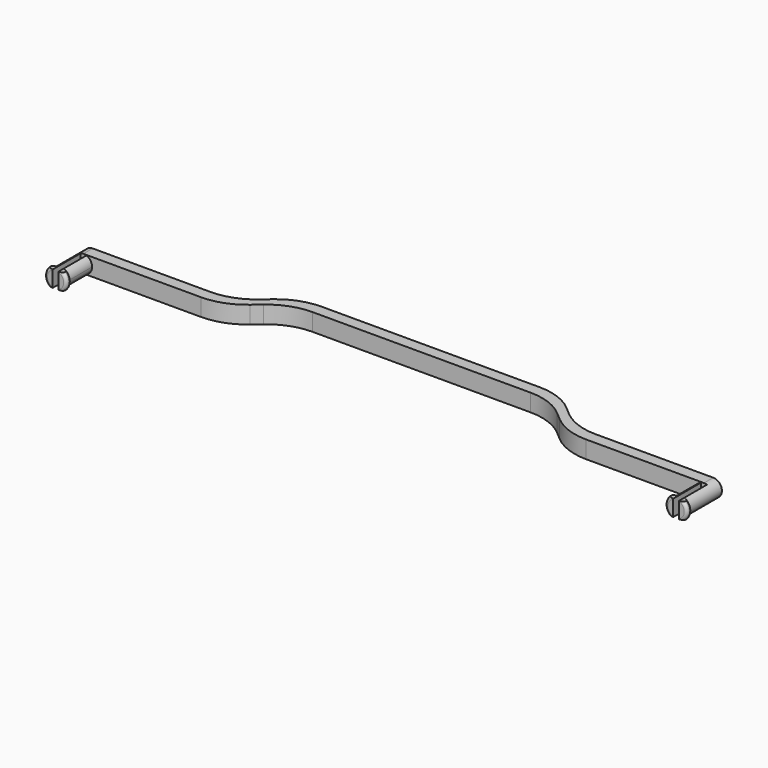
from build123d import *

# Parameters (mm, degrees)
F0_W      = 24
F0_H      = 2
F0_W_2    = 22.5
F1_DEPTH  = 3
F2_R      = 10
F3_R      = 1.5
F4_DEPTH  = 2
F5_DEPTH  = 6
F6_R      = 1.9
F6_R_2    = 1.5
F7_DEPTH  = 1
F9_W      = 1
F9_H      = 3.4420455096
F9_W_2    = 3.6737932861
F9_H_2    = 0.5
F9_W_3    = 2.2944888771
F9_H_3    = 2.8
F9_W_4    = 3.9643547535
F10_DEPTH = 6


# Not quite as in the source:
# - a fillet or chamfer that OpenCascade refuses, or shapes differently, is made with other operations: its cross-section is extruded or revolved along the edge and cut away or added


with BuildPart() as f1:
    # F0 (on Top) → F1 (new body)
    with BuildSketch(Plane.XY):
        with Locations((-41.5, 1)):
            Rectangle(F0_W, F0_H)
        Polygon((-29.5, 2), (-29.5, 0), (-22.5, 6), (-22.5, 8), align=None)
        with Locations((-11.25, 7)):
            Rectangle(F0_W_2, F0_H)
        with Locations((11.25, 7)):
            Rectangle(F0_W_2, F0_H)
        Polygon((22.5, 8), (22.5, 6), (29.5, 0), (29.5, 2), align=None)
        with Locations((41.5, 1)):
            Rectangle(F0_W, F0_H)
    extrude(amount=F1_DEPTH)

    # F2
    f2_edges = [f1.edges().sort_by_distance(p)[0] for p in [
        (-29.5, 2, 1.5),
        (-22.5, 8, 1.5),
        (22.5, 8, 1.5),
        (29.5, 2, 1.5),
        (29.5, 0, 1.5),
        (22.5, 6, 1.5),
        (-22.5, 6, 1.5),
        (-29.5, 0, 1.5),
    ]]
    fillet(f2_edges, radius=F2_R)

    # F3 (on face) → F4 (join, through all)
    with BuildSketch(Plane.XZ):
        with BuildLine():
            Line((-53.5, 0), (-53.5, 3))
            ThreePointArc((-53.5, 3), (-55, 1.5), (-53.5, 0))
        make_face()
        with Locations((53.5, 1.5)):
            Circle(F3_R)
    extrude(amount=-F4_DEPTH)

    # F3 (on face) → F5 (join)
    with BuildSketch(Plane.XZ):
        with BuildLine():
            Line((-53.5, 0), (-53.5, 3))
            ThreePointArc((-53.5, 3), (-55, 1.5), (-53.5, 0))
        make_face()
        with BuildLine():
            ThreePointArc((-53.5, 0), (-52.4393398282, 0.4393398282), (-52, 1.5))
            ThreePointArc((-52, 1.5), (-52.4393398282, 2.5606601718), (-53.5, 3))
            Line((-53.5, 3), (-53.5, 0))
        make_face()
        with Locations((53.5, 1.5)):
            Circle(F3_R)
    extrude(amount=F5_DEPTH)

    # F6 (on face) → F7 (join)
    with BuildSketch(Plane.XZ.offset(6)):
        with Locations((-53.5, 1.5)):
            Circle(F6_R)
        with Locations((-53.5, 1.5)):
            Circle(F6_R_2, mode=Mode.SUBTRACT)
        with Locations((53.5, 1.5)):
            Circle(F6_R)
    extrude(amount=-F7_DEPTH)

    # F8: fillet of radius 0.5 on 4 edges, made by hand

    # F8_s1 → F8_t2 (revolve, cut)
    with BuildSketch(Plane.XY.offset(1.5)):
        with BuildLine():
            ThreePointArc((-51.6, -5.5), (-51.7464466094, -5.8535533906), (-52.1, -6))
            Line((-52.1, -6), (-51.6, -6))
            Line((-51.6, -6), (-51.6, -5.5))
        make_face()
    revolve(axis=Axis((-53.5, -6, 1.5), (0, -1, 0)), mode=Mode.SUBTRACT)

    # F8_s3 → F8_t4 (revolve, cut)
    with BuildSketch(Plane.XY.offset(1.5)):
        with BuildLine():
            ThreePointArc((-52, -5), (-51.7127016654, -5.1736701825), (-51.6, -5.4898979486))
            Line((-51.6, -5.4898979486), (-51.6, -5))
            Line((-51.6, -5), (-52, -5))
        make_face()
    revolve(axis=Axis((-53.5, -5, 1.5), (0, -1, 0)), mode=Mode.SUBTRACT)

    # F8_s5 → F8_t6 (revolve, cut)
    with BuildSketch(Plane.XY.offset(1.5)):
        with BuildLine():
            ThreePointArc((55, -5), (55.2872983346, -5.1736701825), (55.4, -5.4898979486))
            Line((55.4, -5.4898979486), (55.4, -5))
            Line((55.4, -5), (55, -5))
        make_face()
    revolve(axis=Axis((53.5, -5, 1.5), (0, -1, 0)), mode=Mode.SUBTRACT)

    # F8_s7 → F8_t8 (revolve, cut)
    with BuildSketch(Plane.XY.offset(1.5)):
        with BuildLine():
            ThreePointArc((55.4, -5.5), (55.2535533906, -5.8535533906), (54.9, -6))
            Line((54.9, -6), (55.4, -6))
            Line((55.4, -6), (55.4, -5.5))
        make_face()
    revolve(axis=Axis((53.5, -6, 1.5), (0, -1, 0)), mode=Mode.SUBTRACT)

    # F9 (on face) → F10 (cut, through all)
    with BuildSketch(Plane.XZ.offset(6)):
        with Locations((-53.5, -2.1210227548)):
            Rectangle(F9_W, F9_H)
        with Locations((-55.836896643, -0.15)):
            Rectangle(F9_W_2, F9_H_2)
        with Locations((-53.5, -0.15)):
            Rectangle(F9_W, F9_H_2)
        with Locations((-51.8527555615, -0.15)):
            Rectangle(F9_W_3, F9_H_2)
        with Locations((-53.5, 1.5)):
            Rectangle(F9_W, F9_H_3)
        with Locations((-55.9821773767, 3.15)):
            Rectangle(F9_W_4, F9_H_2)
        with Locations((-53.5, 3.15)):
            Rectangle(F9_W, F9_H_2)
        with Locations((-51.8527555615, 3.15)):
            Rectangle(F9_W_3, F9_H_2)
        with Locations((-53.5, 5.1210227548)):
            Rectangle(F9_W, F9_H)
        with Locations((55.836896643, -0.15)):
            Rectangle(F9_W_2, F9_H_2)
        with Locations((53.5, -2.1210227548)):
            Rectangle(F9_W, F9_H)
        with Locations((53.5, -0.15)):
            Rectangle(F9_W, F9_H_2)
        with Locations((53.5, 1.5)):
            Rectangle(F9_W, F9_H_3)
        with Locations((51.8527555615, -0.15)):
            Rectangle(F9_W_3, F9_H_2)
        with Locations((55.9821773767, 3.15)):
            Rectangle(F9_W_4, F9_H_2)
        with Locations((53.5, 3.15)):
            Rectangle(F9_W, F9_H_2)
        with Locations((51.8527555615, 3.15)):
            Rectangle(F9_W_3, F9_H_2)
        with Locations((53.5, 5.1210227548)):
            Rectangle(F9_W, F9_H)
    extrude(amount=-F10_DEPTH, mode=Mode.SUBTRACT)


solid = f1.part
